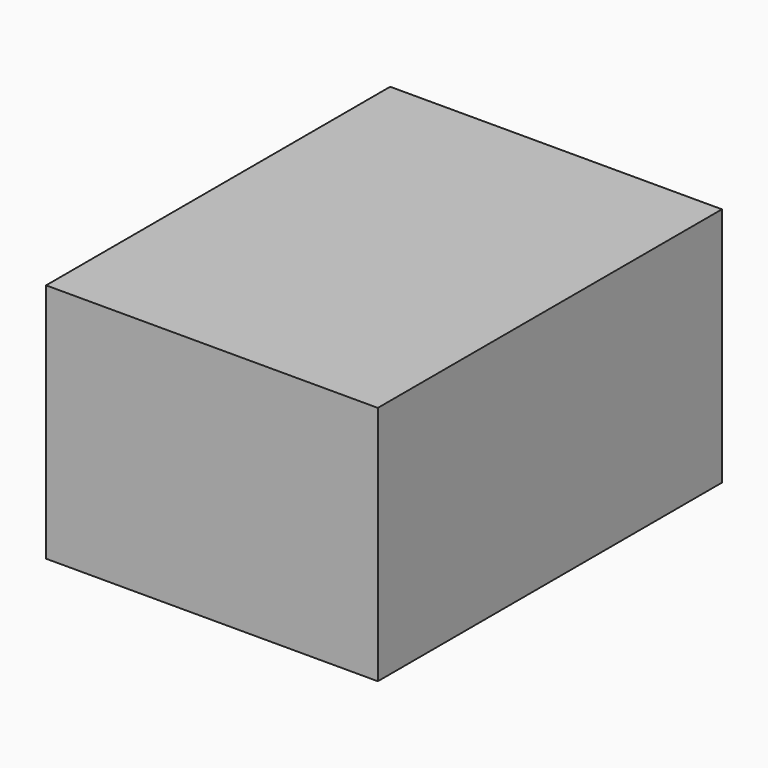
from build123d import *

# Parameters (mm, degrees)
F0_W     = 67.9279565811
F0_H     = 88.0647003651
F1_DEPTH = 49.276


# Not quite as in the source:
# - a feature of the source that left no trace in its solid (it failed there, or was rolled back) is left out


with BuildPart() as f1:
    # F0 (on Top) → F1 (new body)
    with BuildSketch(Plane.XY):
        Rectangle(F0_W, F0_H)
    extrude(amount=-F1_DEPTH)


solid = f1.part
